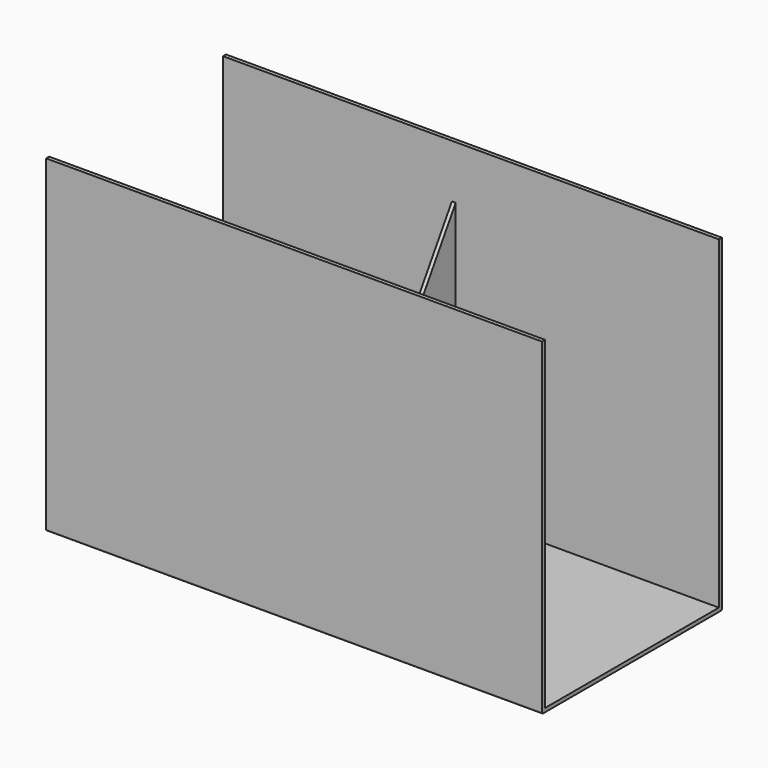
from build123d import *

# Parameters (mm, degrees)
F1_DEPTH = 650
F4_DEPTH = 5
F5_R     = 2


# Not quite as in the source:
# - a feature names something its author has since deleted; it is built from what else it names


with BuildPart() as f1:
    # F0 (on Right) → F1 (new body)
    with BuildSketch(Plane.YZ):
        Polygon((-295, 0), (0, 0), (0, 430), (-5, 430), (-5, 5), (-290, 5), (-290, 430), (-295, 430), align=None)
    extrude(amount=F1_DEPTH)

    # F3 (on offset) → F4 (join)
    with BuildSketch(Plane.YZ.offset(300)):
        Polygon((-230, 0), (-5, 0), (-5, 360), align=None)
    extrude(amount=F4_DEPTH)

    # F5
    f5_edges = [f1.edges().sort_by_distance(p)[0] for p in [
        (325, 0, 0),
        (325, -295, 0),
    ]]
    fillet(f5_edges, radius=F5_R)


solid = f1.part
